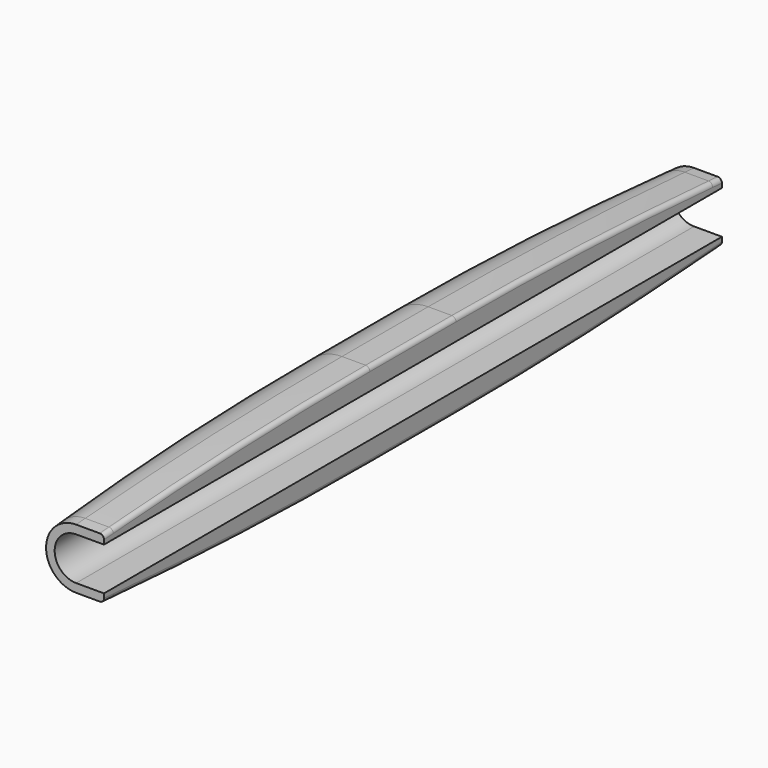
from build123d import *

# Parameters (mm, degrees)
F1_DEPTH    = 180
F2_SIZE2    = 40
F2_SIZE     = 3
F2_2_SIZE2  = 40
F2_2_SIZE   = 3
F3_T1_DEPTH = 100.1185335526
F3_T4_ANGLE = 180
F3_T6_ANGLE = 180
F4_R        = 1


# Not quite as in the source:
# - a fillet or chamfer that OpenCascade refuses, or shapes differently, is made with other operations: its cross-section is extruded or revolved along the edge and cut away or added


with BuildPart() as f1:
    # F0 (on Front) → F1 (new body)
    with BuildSketch(Plane.XZ):
        with BuildLine():
            Line((-6.5, 5), (-2.1602540378, 5))
            Line((-2.1602540378, 5), (0, 5))
            Line((0, 5), (0, 7.5993420768))
            Line((0, 7.5993420768), (0, 10))
            Line((0, 10), (-6.5, 10))
            ThreePointArc((-6.5, 10), (-16.5, 0), (-6.5, -10))
            Line((-6.5, -10), (0, -10))
            Line((0, -10), (0, -7.5993420768))
            Line((0, -7.5993420768), (0, -5))
            Line((0, -5), (-2.1602540378, -5))
            Line((-2.1602540378, -5), (-6.5, -5))
            ThreePointArc((-6.5, -5), (-11.5, 0), (-6.5, 5))
        make_face()
    extrude(amount=F1_DEPTH)

    # F2
    f2_edges = [f1.edges().sort_by_distance(p)[0] for p in [
        (-3.25, -180, 10),
    ]]
    f2_side = f1.faces().sort_by_distance((-11.759278, -180, 0))[0]
    chamfer(f2_edges, length=F2_SIZE, length2=F2_SIZE2, reference=f2_side)

    # F2#2
    f2_2_edges = [f1.edges().sort_by_distance(p)[0] for p in [
        (-3.25, 0, 10),
    ]]
    f2_2_side = f1.faces().sort_by_distance((-11.759278, 0, 0))[0]
    chamfer(f2_2_edges, length=F2_2_SIZE, length2=F2_2_SIZE2, reference=f2_2_side)

    # F3: fillet of radius 1000 on 2 edges, made by hand

    # F3_s2 → F3_t1 (cut)
    with BuildSketch(Plane.YZ.offset(-6.5)):
        with BuildLine():
            ThreePointArc((-102.5525865789, 10), (-139.9737711643, 9.2995821796), (-177.3425348206, 7.1993098885))
            Line((-177.3425348206, 7.1993098885), (-140, 10))
            Line((-140, 10), (-102.5525865789, 10))
        make_face()
        with BuildLine():
            ThreePointArc((-77.4474134211, 10), (-40.0262288357, 9.2995821796), (-2.6574651794, 7.1993098885))
            Line((-2.6574651794, 7.1993098885), (-40, 10))
            Line((-40, 10), (-77.4474134211, 10))
        make_face()
        with BuildLine():
            ThreePointArc((-2.6574651794, -7.1993098885), (-40.0262288357, -9.2995821796), (-77.4474134211, -10))
            Line((-77.4474134211, -10), (-40, -10))
            Line((-40, -10), (-2.6574651794, -7.1993098885))
        make_face()
        with BuildLine():
            ThreePointArc((-177.3425348206, -7.1993098885), (-139.9737711643, -9.2995821796), (-102.5525865789, -10))
            Line((-102.5525865789, -10), (-140, -10))
            Line((-140, -10), (-177.3425348206, -7.1993098885))
        make_face()
    extrude(amount=F3_T1_DEPTH, mode=Mode.SUBTRACT)

    # F3_s3 → F3_t4 (revolve, cut)
    with BuildSketch(Plane.YZ.offset(-6.5)):
        with BuildLine():
            ThreePointArc((-77.4474134211, 10), (-40.0262288357, 9.2995821796), (-2.6574651794, 7.1993098885))
            Line((-2.6574651794, 7.1993098885), (-40, 10))
            Line((-40, 10), (-77.4474134211, 10))
        make_face()
    revolve(axis=Axis((-6.5, -40, 0), (0, -1, 0)), revolution_arc=F3_T4_ANGLE, mode=Mode.SUBTRACT)

    # F3_s5 → F3_t6 (revolve, cut)
    with BuildSketch(Plane.YZ.offset(-6.5)):
        with BuildLine():
            ThreePointArc((-102.5525865789, 10), (-139.9737711643, 9.2995821796), (-177.3425348206, 7.1993098885))
            Line((-177.3425348206, 7.1993098885), (-140, 10))
            Line((-140, 10), (-102.5525865789, 10))
        make_face()
    revolve(axis=Axis((-6.5, -140, 0), (0, -1, 0)), revolution_arc=F3_T6_ANGLE, mode=Mode.SUBTRACT)

    # F4
    f4_edges = [f1.edges().sort_by_distance(p)[0] for p in [
        (0, -90, 10),
        (0, -90, -10),
    ]]
    fillet(f4_edges, radius=F4_R)


solid = f1.part
